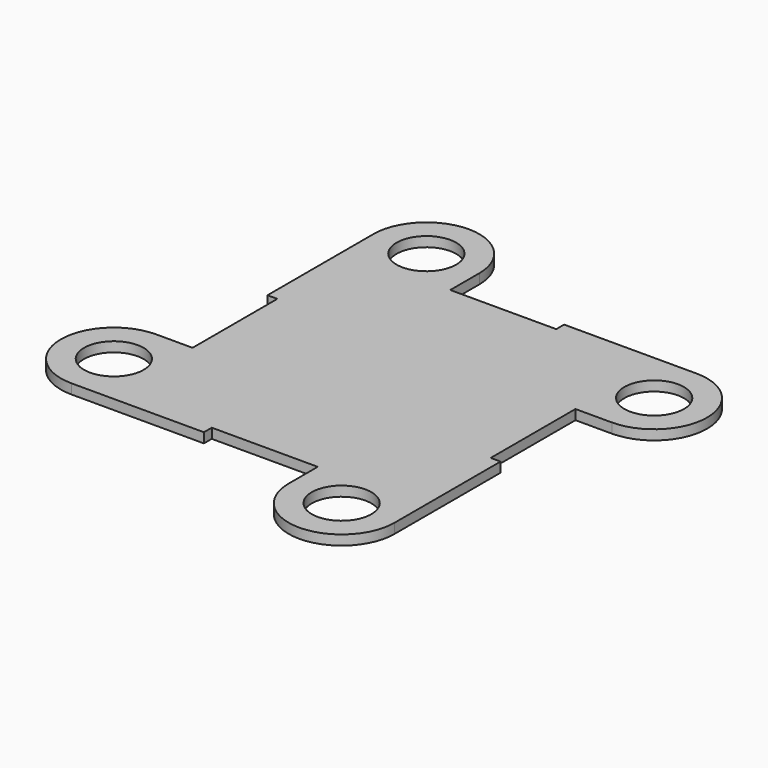
from build123d import *

# Parameters (mm, degrees)
F0_W            = 76.2
F0_H            = 76.2
F1_DEPTH        = 2.3622
F2_W            = 25.4
F2_H            = 2.3622
F4_DEPTH        = 25.4
F4_COPIES_COUNT = 4
F6_DEPTH        = 2.3622
F6_COPIES_COUNT = 4
F7_R            = 7.14375
F8_DEPTH        = 2.3632
F8_COPIES_COUNT = 4


# Not quite as in the source:
# - a pattern or mirror of a feature is missing from the dataset's text; its kind, count and spacing are read off the source's solid


with BuildPart() as f1:
    # F0 (on Top) → F1 (new body)
    with BuildSketch(Plane.XY):
        Rectangle(F0_W, F0_H)
    extrude(amount=F1_DEPTH)

    # F2 (on face) → F4 (cut)
    with BuildSketch(Plane.XY.offset(2.3622)):
        with Locations((0, 36.9189)):
            Rectangle(F2_W, F2_H)
    f4 = extrude(amount=-F4_DEPTH, mode=Mode.SUBTRACT)

    # F4_copies: F4 ×4 about axis
    f4_copies_axis = Axis((0, 0, 0), (0, 0, 1))
    for i in range(1, F4_COPIES_COUNT):
        add(f4.rotate(f4_copies_axis, i * 360 / F4_COPIES_COUNT), mode=Mode.SUBTRACT)

    # F5 (on face) → F6 (join, through all)
    with BuildSketch(Plane.XY.offset(2.3622)):
        with BuildLine():
            Line((-38.1, 44.45), (-38.1, 38.1))
            Line((-38.1, 38.1), (-12.7, 38.1))
            Line((-12.7, 38.1), (-12.7, 44.45))
            ThreePointArc((-12.7, 44.45), (-25.4, 57.15), (-38.1, 44.45))
        make_face()
    f6 = extrude(amount=-F6_DEPTH)

    # F6_copies: F6 ×4 about axis
    f6_copies_axis = Axis((0, 0, 0), (0, 0, 1))
    for i in range(1, F6_COPIES_COUNT):
        add(f6.rotate(f6_copies_axis, i * 360 / F6_COPIES_COUNT))

    # F7 (on Top) → F8 (cut, through all)
    with BuildSketch(Plane.XY):
        with Locations((-25.4, 44.45)):
            Circle(F7_R)
    f8 = extrude(amount=F8_DEPTH, mode=Mode.SUBTRACT)

    # F8_copies: F8 ×4 about axis
    f8_copies_axis = Axis((0, 0, 0), (0, 0, 1))
    for i in range(1, F8_COPIES_COUNT):
        add(f8.rotate(f8_copies_axis, i * 360 / F8_COPIES_COUNT), mode=Mode.SUBTRACT)


solid = f1.part
